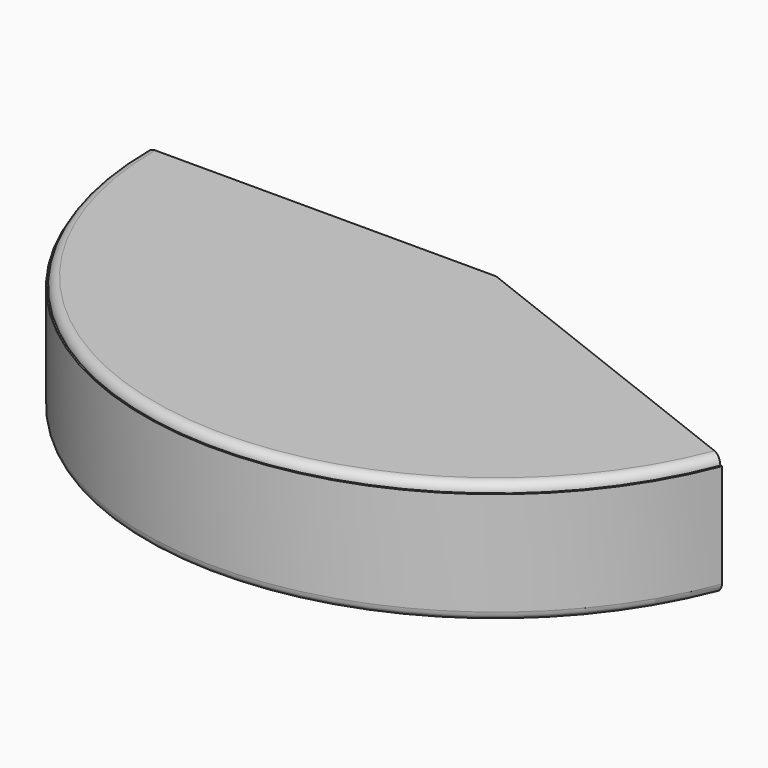
from build123d import *

# Parameters (mm, degrees)
F0_R         = 39
F0_R_2       = 38.1
F1_DEPTH     = 9
F2_DEPTH     = 10
F0_W         = 32
F0_H         = 32
F3_DEPTH     = 2.5
F5_R         = 38.8254389769
F6_DEPTH     = 2
F7_R         = 0.99999
F9_DEPTH     = 12.5
F10_DEPTH    = 12.5
F11_DEPTH    = 2.5
F12_T2_ANGLE = 166.0974661722
F13_DEPTH    = 14
F14_R        = 0.5


# Not quite as in the source:
# - a fillet or chamfer that OpenCascade refuses, or shapes differently, is made with other operations: its cross-section is extruded or revolved along the edge and cut away or added
# - a fillet or chamfer is up to 0.001 mm smaller than in the source, because OpenCascade refuses the exact size


with BuildPart() as f1:
    # F0 (on Top) → F1 (new body)
    with BuildSketch(Plane.XY):
        Circle(F0_R)
        Circle(F0_R_2, mode=Mode.SUBTRACT)
    extrude(amount=F1_DEPTH)

    # F0 (on Top) → F2 (join)
    with BuildSketch(Plane.XY):
        Circle(F0_R)
        Circle(F0_R_2, mode=Mode.SUBTRACT)
    extrude(amount=F2_DEPTH)

    # F5 (on offset) → F6 (join)
    with BuildSketch(Plane.XY.offset(9)):
        Circle(F5_R)
    extrude(amount=F6_DEPTH)

    # F7 (radius 1 in the source; OpenCascade refuses exactly that, so slightly less here)
    f7_edges = [f1.edges().sort_by_distance(p)[0] for p in [
        (-38.825439, 0, 11),
    ]]
    fillet(f7_edges, radius=F7_R)


with BuildPart() as f3:
    # F0 (on Top) → F3 (new body)
    with BuildSketch(Plane.XY):
        Circle(F0_R_2)
        Rectangle(F0_W, F0_H, mode=Mode.SUBTRACT)
    extrude(amount=-F3_DEPTH)


with BuildPart() as f9:
    # F8 (on Top) → F9 (new body, symmetric)
    with BuildSketch(Plane.XY):
        Polygon((-41.2051826715, 48.0051673949), (-42.0097357945, 0), (0, 0), (36.1852608621, -14.1163477674), (49.7808791697, -14.1163477674), (49.2908842862, 48.0051673949), align=None)
    extrude(amount=F9_DEPTH, both=True)


with BuildPart() as f10_tool:
    # F8 (on Top) → F10 (new body, symmetric)
    with BuildSketch(Plane.XY):
        Polygon((-41.2051826715, 48.0051673949), (-42.0097357945, 0), (0, 0), (36.1852608621, -14.1163477674), (49.7808791697, -14.1163477674), (49.2908842862, 48.0051673949), align=None)
    extrude(amount=F10_DEPTH, both=True)


with BuildPart() as f1_1:
    add(f1.part)

    # F10: cut by f10_tool
    add(f10_tool.part, mode=Mode.SUBTRACT)


with BuildPart() as f3_1:
    add(f3.part)

    # F10: cut by f10_tool
    add(f10_tool.part, mode=Mode.SUBTRACT)


with BuildPart() as f9_1:
    add(f9.part)

    # F10: cut by f10_tool
    add(f10_tool.part, mode=Mode.SUBTRACT)


with BuildPart() as f11:
    # F11 (new): a face of the model
    f11_faces = [f1_1.part.faces().sort_by_distance(p)[0] for p in [
        (-38.55, -0.8484965841, 0),
    ]]
    extrude(f11_faces, amount=F11_DEPTH)

    # F12: fillet of radius 1 on 1 edges, made by hand

    # F12_s1 → F12_t2 (revolve, cut)
    with BuildSketch(Plane(origin=(0, 0, 0), x_dir=(0, 0, 1), z_dir=(0.0638176413, 0.9979615767, 0))):
        with BuildLine():
            ThreePointArc((-1.5050125629, -39), (-2.1758329561, -38.7416198487), (-2.5, -38.1))
            Line((-2.5, -38.1), (-2.5, -39))
            Line((-2.5, -39), (-1.5050125629, -39))
        make_face()
    revolve(axis=Axis((0, 0, -2.5), (0, 0, 1)), revolution_arc=F12_T2_ANGLE, mode=Mode.SUBTRACT)


with BuildPart() as f1_2:
    add(f1_1.part)

    # F13 (add): a face of the model
    f13_faces = [f3_1.part.faces().sort_by_distance(p)[0] for p in [
        (-27.05, 0, -1.25),
    ]]

    add(f3_1.part)  # F13 merges F3

    add(f11.part)  # F13 merges F11
    extrude(f13_faces, amount=F13_DEPTH)

    # F14
    f14_edges = [f1_2.edges().sort_by_distance(p)[0] for p in [
        (-27.05, 14, -2.5),
        (-27.05, 14, 0),
    ]]
    fillet(f14_edges, radius=F14_R)


solid = f1_2.part
